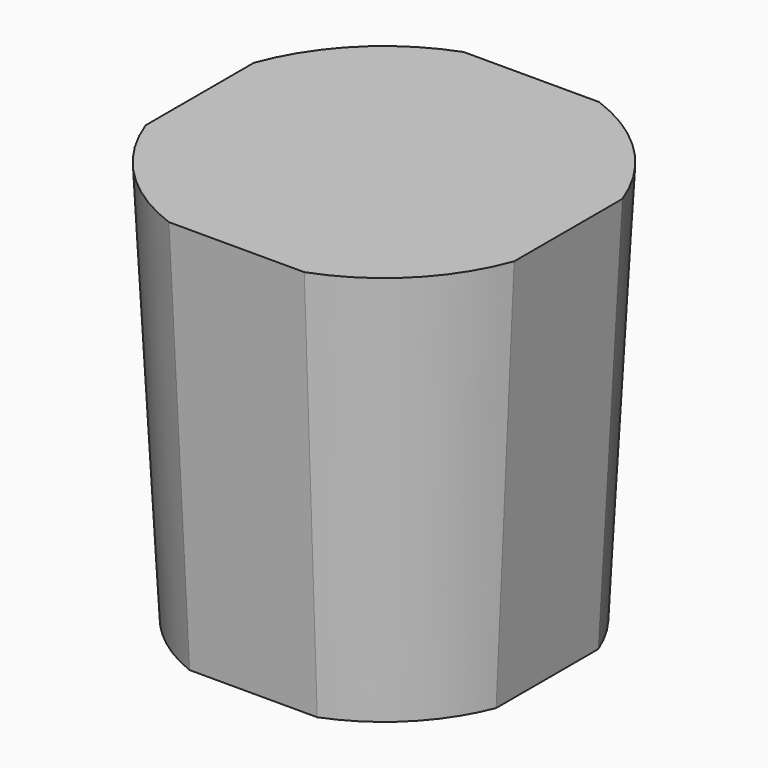
from build123d import *

# Parameters (mm, degrees)
F1_DEPTH               = 80
DRAFT_F1_DRAFTED_ANGLE = -3


# Not quite as in the source:
# - an extrude with a draft is written as a straight extrude whose walls are then drafted


with BuildPart() as f1:
    # F0 (on Top) → F1 (new body)
    with BuildSketch(Plane.XY):
        with BuildLine():
            Line((12.7101272713, 32.5), (-12.7101272713, 32.5))
            ThreePointArc((-12.7101272713, 32.5), (-24.6758721756, 24.6758721756), (-32.5, 12.7101272713))
            Line((-32.5, 12.7101272713), (-32.5, -12.7101272713))
            ThreePointArc((-32.5, -12.7101272713), (-24.6758721756, -24.6758721756), (-12.7101272713, -32.5))
            Line((-12.7101272713, -32.5), (12.7101272713, -32.5))
            ThreePointArc((12.7101272713, -32.5), (24.6758721756, -24.6758721756), (32.5, -12.7101272713))
            Line((32.5, -12.7101272713), (32.5, 12.7101272713))
            ThreePointArc((32.5, 12.7101272713), (24.6758721756, 24.6758721756), (12.7101272713, 32.5))
        make_face()
    extrude(amount=F1_DEPTH)

    # draft_F1_drafted
    draft_f1_drafted_walls = [f1.faces().sort_by_distance(p)[0] for p in [
        (24.6758721756, 24.6758721756, 53.3333333333),
        (0, 32.5, 53.3333333333),
        (-24.6758721756, 24.6758721756, 53.3333333333),
        (-32.5, 0, 53.3333333333),
        (-24.6758721756, -24.6758721756, 53.3333333333),
        (0, -32.5, 53.3333333333),
        (24.6758721756, -24.6758721756, 53.3333333333),
        (32.5, 0, 53.3333333333),
    ]]
    draft(draft_f1_drafted_walls, neutral_plane=Plane.XY, angle=DRAFT_F1_DRAFTED_ANGLE)


solid = f1.part
